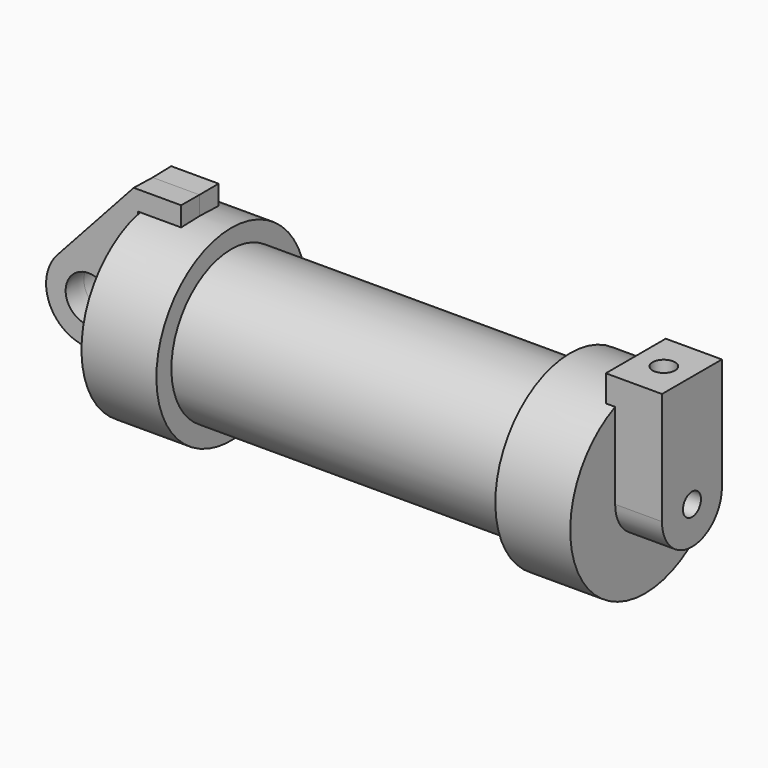
from build123d import *

# Parameters (mm, degrees)
F0_W      = 5.842
F0_H      = 12.7
F0_R      = 3.175
F2_DEPTH  = 3.175
F2_TAPER  = -1
F4_DEPTH  = 1.27
F3_R      = 1.524
F5_DEPTH  = 6.35
F6_R      = 1.524
F7_DEPTH  = 6.35
F10_R     = 1.524
F11_DEPTH = 10.414


# Not quite as in the source:
# - a feature of the source that left no trace in its solid (it failed there, or was rolled back) is left out


with BuildPart() as f1:
    # F0 (on Front) → F1 (revolve)
    with BuildSketch(Plane.XZ):
        Polygon((5.842, 12.7), (5.842, 0), (66.294, 0), (66.294, 12.7), (56.134, 12.7), (56.134, 10.16), (10.16, 10.16), (10.16, 12.7), align=None)
        with Locations((2.921, 6.35)):
            Rectangle(F0_W, F0_H)
    revolve(axis=Axis((33.147, 0, 0), (-1, 0, 0)))

    # F0 (on Front) → F2 (join, symmetric)
    with BuildSketch(Plane.XZ):
        with BuildLine():
            Line((5.842, 0), (0, 0))
            Line((0, 0), (-0.9398, 0))
            ThreePointArc((-0.9398, 0), (-3.1957909266, -4.5493385486), (-8.1826630726, -5.5069827884))
            Line((-8.1826630726, -5.5069827884), (5.842, -9.398))
            Line((5.842, -9.398), (5.842, 0))
        make_face()
        with BuildLine():
            ThreePointArc((-8.1826630726, -5.5069827884), (-3.1957909266, -4.5493385486), (-0.9398, 0))
            ThreePointArc((-0.9398, 0), (-4.5919612295, 5.3297205562), (-10.8806298187, 3.8475430269))
            ThreePointArc((-10.8806298187, 3.8475430269), (-12.1459778134, -1.5837270034), (-8.1826630726, -5.5069827884))
        make_face()
        with Locations((-6.6548, 0)):
            Circle(F0_R, mode=Mode.SUBTRACT)
        with BuildLine():
            Line((-0.9398, 0), (0, 0))
            Line((0, 0), (0, 12.7))
            Line((0, 12.7), (5.842, 12.7))
            Line((5.842, 12.7), (5.842, 15.24))
            Line((5.842, 15.24), (-0.508, 15.24))
            Line((-0.508, 15.24), (-10.8806298187, 3.8475430269))
            ThreePointArc((-10.8806298187, 3.8475430269), (-4.5919612295, 5.3297205562), (-0.9398, 0))
        make_face()
    extrude(amount=F2_DEPTH, both=True, taper=F2_TAPER)

    # F3 (on face) → F4 (join)
    with BuildSketch(Plane.YZ.offset(66.294)):
        with BuildLine():
            ThreePointArc((-5.08, 11.6397422652), (0, 12.7), (5.08, 11.6397422652))
            Line((5.08, 11.6397422652), (5.08, 15.24))
            Line((5.08, 15.24), (-5.08, 15.24))
            Line((-5.08, 15.24), (-5.08, 11.6397422652))
        make_face()
    extrude(amount=-F4_DEPTH)

    # F3 (on face) → F5 (join)
    with BuildSketch(Plane.YZ.offset(66.294)):
        with BuildLine():
            ThreePointArc((-5.08, 11.6397422652), (0, 12.7), (5.08, 11.6397422652))
            Line((5.08, 11.6397422652), (5.08, 15.24))
            Line((5.08, 15.24), (-5.08, 15.24))
            Line((-5.08, 15.24), (-5.08, 11.6397422652))
        make_face()
        with BuildLine():
            ThreePointArc((-5.08, 0), (0, 5.08), (5.08, 0))
            Line((5.08, 0), (5.08, 11.6397422652))
            ThreePointArc((5.08, 11.6397422652), (0, 12.7), (-5.08, 11.6397422652))
            Line((-5.08, 11.6397422652), (-5.08, 0))
        make_face()
        with BuildLine():
            ThreePointArc((-5.08, 0), (0, -5.08), (5.08, 0))
            ThreePointArc((5.08, 0), (0, 5.08), (-5.08, 0))
        make_face()
        Circle(F3_R, mode=Mode.SUBTRACT)
        Circle(F3_R)
    extrude(amount=F5_DEPTH)

    # F6 (on face) → F7 (cut, through all)
    with BuildSketch(Plane.YZ.offset(72.644)):
        Circle(F6_R)
    extrude(amount=-F7_DEPTH, mode=Mode.SUBTRACT)

    # F10 (on face) → F11 (cut)
    with BuildSketch(Plane.XY.offset(15.24)):
        with Locations((68.834, 0)):
            Circle(F10_R)
    extrude(amount=-F11_DEPTH, mode=Mode.SUBTRACT)


solid = f1.part
